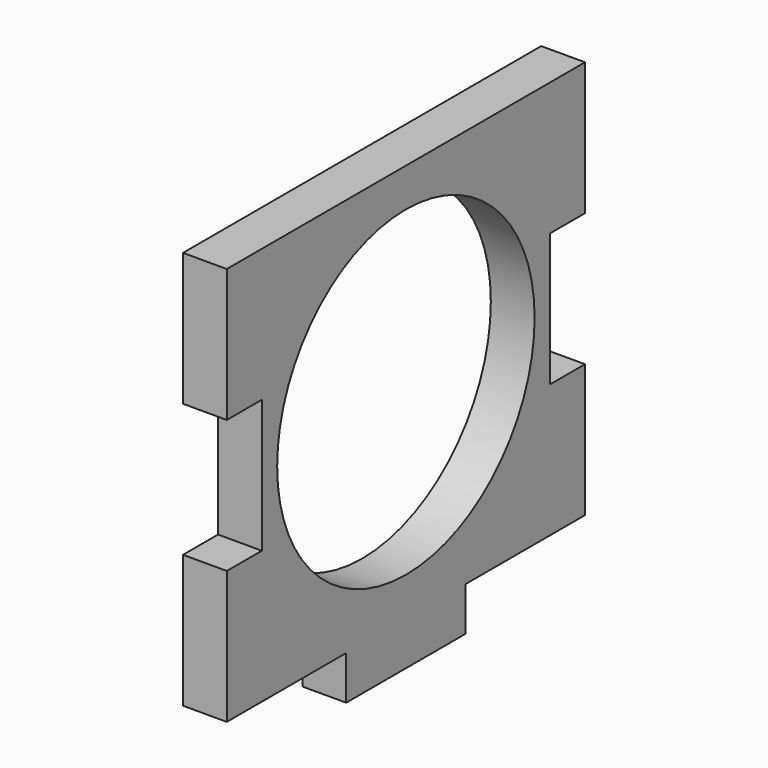
from build123d import *

# Parameters (mm, degrees)
F1_DEPTH = 19.05
F2_D     = 139.999974
F2_DEPTH = 50.8
F2_TIP   = 42.0602355207


with BuildPart() as f1:
    # F0 (on Right) → F1 (new body)
    with BuildSketch(Plane.YZ):
        Polygon((110.4406434166, 38.438666836), (110.4406434166, 96.266), (-84.3773565834, 96.266), (-84.3773565834, 38.438666836), (-65.3273565834, 38.438666836), (-65.3273565834, -19.388666836), (-84.3773565834, -19.388666836), (-84.3773565834, -77.216), (-19.4380147834, -77.216), (-19.4380147834, -96.266), (45.5013016166, -96.266), (45.5013016166, -77.216), (110.4406434166, -77.216), (110.4406434166, -19.388666836), (91.3906434166, -19.388666836), (91.3906434166, 38.438666836), align=None)
    extrude(amount=F1_DEPTH)

    # F2
    with Locations(Plane(origin=(0, 0, 0), x_dir=(0, 1, 0), z_dir=(-1, 0, 0))):
        with Locations((13.0316434166, -9.525)):
            Hole(F2_D / 2, depth=F2_DEPTH)
            with Locations((0, 0, -(F2_DEPTH + F2_TIP / 2))):  # 118° drill point
                Cone(0, F2_D / 2, F2_TIP, mode=Mode.SUBTRACT)


solid = f1.part
